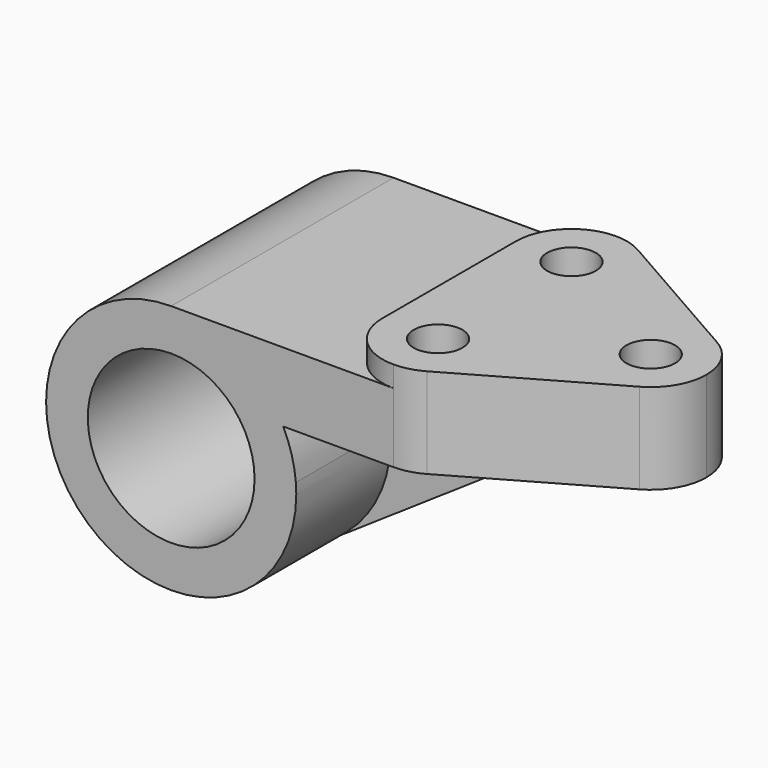
from build123d import *
from build123d import SkipClean  # not in build123d's __all__

# Parameters (mm, degrees)
F0_R     = 5.5626
F1_DEPTH = 20.6502
F2_DEPTH = 15.875
F4_DEPTH = 31.75
F6_DEPTH = 4.7625
F8_DEPTH = 381


with BuildPart() as f1:
    # F0 (on Top) → F1 (new body)
    with BuildSketch(Plane.XY):
        with BuildLine():
            ThreePointArc((6.2991554441, -11.0277214642), (-12.7, 0), (6.2991554441, 11.0277214642))
            Line((6.2991554441, 11.0277214642), (-27.0510445559, 30.0777214642))
            ThreePointArc((-27.0510445559, 30.0777214642), (-22.3663647377, 25.4253715915), (-20.6502, 19.05))
            ThreePointArc((-20.6502, 19.05), (-33.3502, 6.35), (-46.0502, 19.05))
            Line((-46.0502, 19.05), (-46.0502, -19.05))
            ThreePointArc((-46.0502, -19.05), (-33.3502, -6.35), (-20.6502, -19.05))
            ThreePointArc((-20.6502, -19.05), (-22.3663647377, -25.4253715915), (-27.0510445559, -30.0777214642))
            Line((-27.0510445559, -30.0777214642), (6.2991554441, -11.0277214642))
        make_face()
        with BuildLine():
            ThreePointArc((-20.6502, 19.05), (-22.3663647377, 25.4253715915), (-27.0510445559, 30.0777214642))
            ThreePointArc((-27.0510445559, 30.0777214642), (-30.0915240875, 31.3248128824), (-33.3502, 31.75))
            ThreePointArc((-33.3502, 31.75), (-42.3304561211, 28.0302561211), (-46.0502, 19.05))
            ThreePointArc((-46.0502, 19.05), (-33.3502, 6.35), (-20.6502, 19.05))
        make_face()
        with Locations((-33.3502, 19.05)):
            Circle(F0_R, mode=Mode.SUBTRACT)
        with BuildLine():
            ThreePointArc((6.2991554441, -11.0277214642), (10.9838352623, -6.3753715915), (12.7, 0))
            ThreePointArc((12.7, 0), (10.9838352623, 6.3753715915), (6.2991554441, 11.0277214642))
            ThreePointArc((6.2991554441, 11.0277214642), (-12.7, 0), (6.2991554441, -11.0277214642))
        make_face()
        Circle(F0_R, mode=Mode.SUBTRACT)
        with BuildLine():
            ThreePointArc((-33.3502, -31.75), (-30.0915240875, -31.3248128824), (-27.0510445559, -30.0777214642))
            ThreePointArc((-27.0510445559, -30.0777214642), (-22.3663647377, -25.4253715915), (-20.6502, -19.05))
            ThreePointArc((-20.6502, -19.05), (-33.3502, -6.35), (-46.0502, -19.05))
            ThreePointArc((-46.0502, -19.05), (-42.3304561211, -28.0302561211), (-33.3502, -31.75))
        make_face()
        with Locations((-33.3502, -19.05)):
            Circle(F0_R, mode=Mode.SUBTRACT)
    extrude(amount=F1_DEPTH)

    # F0 (on Top) → F2 (join)
    with BuildSketch(Plane.XY):
        with BuildLine():
            ThreePointArc((-46.0502, 19.05), (-42.3304561211, 28.0302561211), (-33.3502, 31.75))
            Line((-33.3502, 31.75), (-84.1502, 31.75))
            Line((-84.1502, 31.75), (-84.1502, -31.75))
            Line((-84.1502, -31.75), (-33.3502, -31.75))
            ThreePointArc((-33.3502, -31.75), (-42.3304561211, -28.0302561211), (-46.0502, -19.05))
            Line((-46.0502, -19.05), (-46.0502, 19.05))
        make_face()
    extrude(amount=F2_DEPTH)

    # F3 (on Front) → F4 (join, symmetric)
    with BuildSketch(Plane.XZ):
        with BuildLine():
            ThreePointArc((-55.6745916055, -10.31875), (-56.6256842933, -5.0233040887), (-58.5525316492, 0))
            Line((-58.5525316492, 0), (-69.9511683429, 0))
            ThreePointArc((-69.9511683429, 0), (-66.3542165618, -5.9025391898), (-65.1002, -12.7))
            ThreePointArc((-65.1002, -12.7), (-97.6205841816, -26.1703841816), (-84.1502, 6.35))
            Line((-84.1502, 6.35), (-84.1502, 15.875))
            ThreePointArc((-84.1502, 15.875), (-104.3557762724, -32.9055762724), (-55.5752, -12.7))
            ThreePointArc((-55.5752, -12.7), (-55.6000587142, -11.5083383184), (-55.6745916055, -10.31875))
        make_face()
    extrude(amount=F4_DEPTH, both=True)

    # F5 (on Front) → F6 (join, symmetric)
    with BuildSketch(Plane.XZ):
        with BuildLine():
            ThreePointArc((-58.5525316492, 0), (-56.5215204273, -19.9929205446), (-68.1551747025, -36.3788891364))
            Line((-68.1551747025, -36.3788891364), (-14.3002, 0))
            Line((-14.3002, 0), (-58.5525316492, 0))
        make_face()
    extrude(amount=F6_DEPTH, both=True)

    # F7 (on face) → F8 (cut, symmetric)
    with BuildSketch(Plane.XZ.offset(31.75)):
        with BuildLine():
            ThreePointArc((-69.9511683429, 0), (-76.3730700667, 4.6901912008), (-84.1502, 6.35))
            ThreePointArc((-84.1502, 6.35), (-97.6205841816, -26.1703841816), (-65.1002, -12.7))
            ThreePointArc((-65.1002, -12.7), (-66.3542165618, -5.9025391898), (-69.9511683429, 0))
        make_face()
    with SkipClean():  # cleaning this boolean's faces spoils the solid; the shape is the same uncleaned
        extrude(amount=F8_DEPTH, both=True, mode=Mode.SUBTRACT)


solid = f1.part
